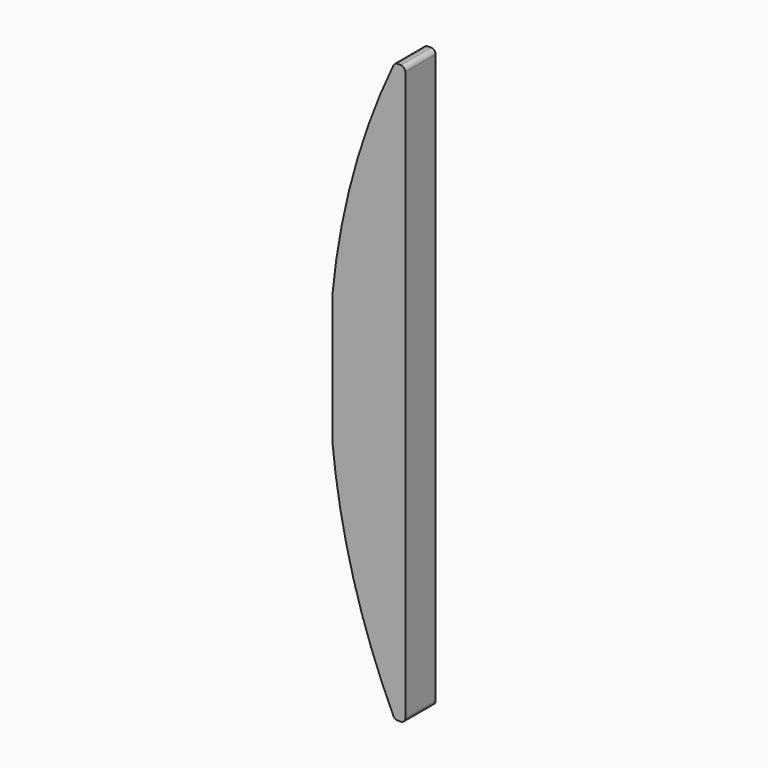
from build123d import *

# Parameters (mm, degrees)
F1_DEPTH    = 25
F2_T1_DEPTH = 34.5185252635
F2_T3_DEPTH = 40
F2_T5_DEPTH = 25.7185484132


# Not quite as in the source:
# - a fillet or chamfer that OpenCascade refuses, or shapes differently, is made with other operations: its cross-section is extruded or revolved along the edge and cut away or added


with BuildPart() as f1:
    # F0 (on Front) → F1 (new body)
    with BuildSketch(Plane.XZ):
        with BuildLine():
            Line((-7, 0), (0, 0))
            Line((0, 0), (0, 380))
            Line((0, 380), (-7, 380))
            ThreePointArc((-7, 380), (-33.9910126529, 307.7803129177), (-48, 231.9651017804))
            Line((-48, 231.9651017804), (-48, 190))
            Line((-48, 190), (-48, 148.0348982196))
            ThreePointArc((-48, 148.0348982196), (-33.9910126529, 72.2196870823), (-7, 0))
        make_face()
    extrude(amount=F1_DEPTH)

    # F2: fillet of radius 3 on 5 edges, made by hand

    # F2_s2 → F2_t1 (cut)
    with BuildSketch(Plane.XZ.offset(-4.7592626318)):
        with BuildLine():
            ThreePointArc((-7.8159850821, 378.2800403279), (-6.7089962565, 379.533783829), (-5.1027772465, 380))
            Line((-5.1027772465, 380), (-7, 380))
            ThreePointArc((-7, 380), (-7.408920068, 379.1404602023), (-7.8159850821, 378.2800403279))
        make_face()
        with BuildLine():
            ThreePointArc((-7.8159850821, 1.7199596721), (-6.7089962565, 0.466216171), (-5.1027772465, 0))
            Line((-5.1027772465, 0), (-7, 0))
            ThreePointArc((-7, 0), (-7.408920068, 0.8595397977), (-7.8159850821, 1.7199596721))
        make_face()
    extrude(amount=F2_T1_DEPTH, mode=Mode.SUBTRACT)

    # F2_s4 → F2_t3 (cut)
    with BuildSketch(Plane.XZ.offset(-7.5)):
        with BuildLine():
            ThreePointArc((-3, 380), (-0.8786796564, 379.1213203436), (0, 377))
            Line((0, 377), (0, 380))
            Line((0, 380), (-3, 380))
        make_face()
        with BuildLine():
            ThreePointArc((0, 3), (-0.8786796564, 0.8786796564), (-3, 0))
            Line((-3, 0), (0, 0))
            Line((0, 0), (0, 3))
        make_face()
    extrude(amount=F2_T3_DEPTH, mode=Mode.SUBTRACT)

    # F2_s6 → F2_t5 (cut)
    with BuildSketch(Plane.XZ.offset(-0.3592742066)):
        with BuildLine():
            ThreePointArc((-47.9863097291, 232.1081578861), (-47.9965754777, 231.9651832447), (-48, 231.8218814431))
            Line((-48, 231.8218814431), (-48, 231.9651017804))
            ThreePointArc((-48, 231.9651017804), (-47.9931606883, 232.0366303906), (-47.9863097291, 232.1081578861))
        make_face()
    extrude(amount=F2_T5_DEPTH, mode=Mode.SUBTRACT)


solid = f1.part
